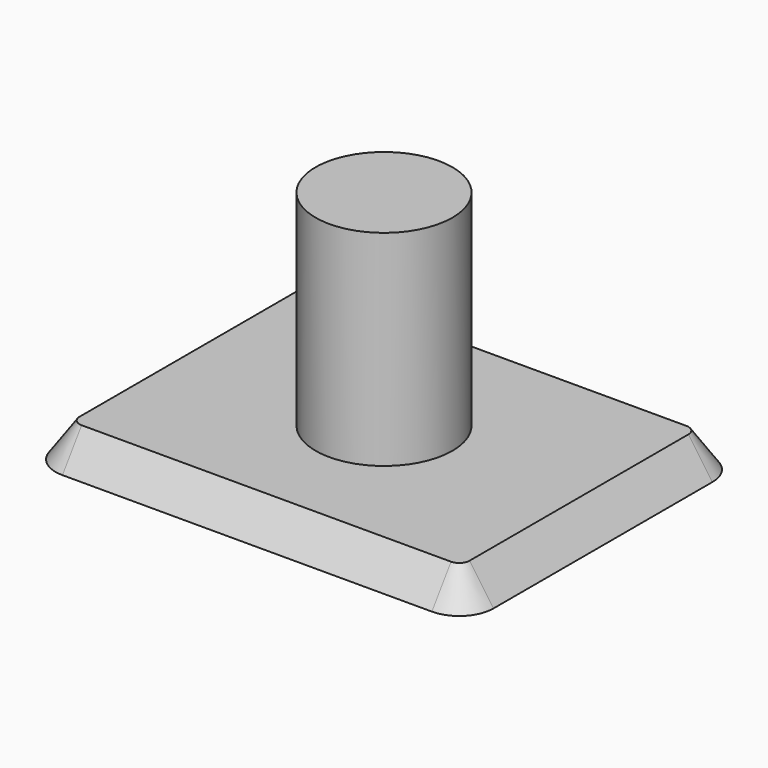
from build123d import *

# Parameters (mm, degrees)
F0_W     = 32
F0_H     = 25
F0_R     = 5
F1_DEPTH = 2.5
F2_R     = 2.5
F3_SIZE2 = 2.49999
F3_SIZE  = 1.750509
F4_DEPTH = 17.5


# Not quite as in the source:
# - a fillet or chamfer is up to 0.001 mm smaller than in the source, because OpenCascade refuses the exact size


with BuildPart() as f1:
    # F0 (on Top) → F1 (new body)
    with BuildSketch(Plane.XY):
        Rectangle(F0_W, F0_H)
        Circle(F0_R, mode=Mode.SUBTRACT)
    extrude(amount=F1_DEPTH)

    # F2
    f2_edges = [f1.edges().sort_by_distance(p)[0] for p in [
        (-16, -12.5, 1.25),
        (16, -12.5, 1.25),
        (16, 12.5, 1.25),
        (-16, 12.5, 1.25),
    ]]
    fillet(f2_edges, radius=F2_R)

    # F3 (size 1.7505188455 and 2.5 in the source; OpenCascade refuses exactly that, so slightly less here)
    f3_edges = [f1.edges().sort_by_distance(p)[0] for p in [
        (0, -12.5, 2.5),
        (-16, 0, 2.5),
        (15.267767, -11.767767, 2.5),
        (16, 0, 2.5),
        (15.267767, 11.767767, 2.5),
        (0, 12.5, 2.5),
        (-15.267767, 11.767767, 2.5),
        (-15.267767, -11.767767, 2.5),
    ]]
    f3_side = f1.faces().sort_by_distance((0, 12.093921, 2.5))[0]
    chamfer(f3_edges, length=F3_SIZE, length2=F3_SIZE2, reference=f3_side)

    # F0 (on Top) → F4 (join)
    with BuildSketch(Plane.XY):
        Circle(F0_R)
    extrude(amount=F4_DEPTH)


solid = f1.part
